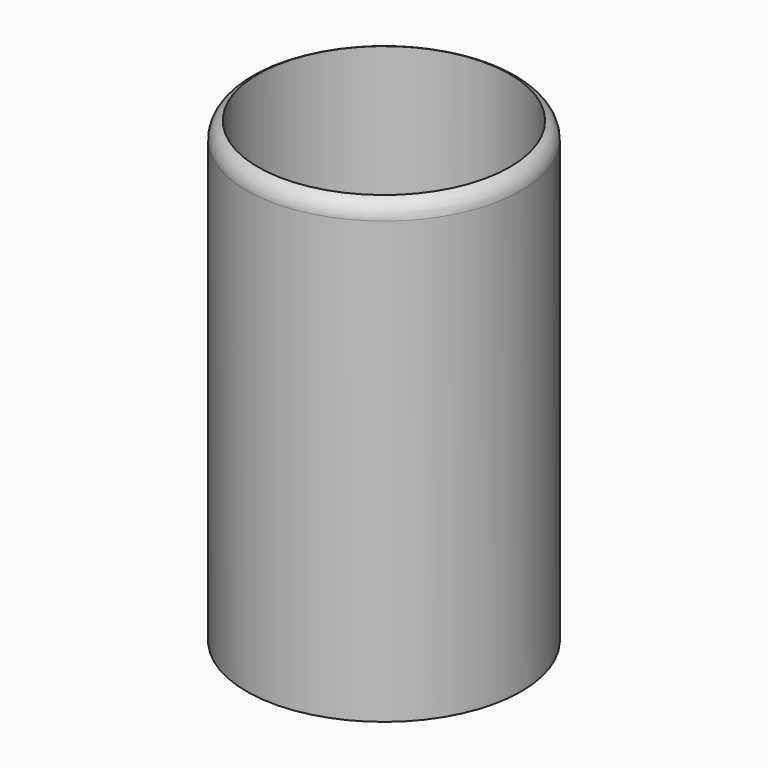
from build123d import *

# Parameters (mm, degrees)
F0_R     = 38.1
F0_R_2   = 34.925
F1_DEPTH = 127
F2_R     = 34.925
F3_DEPTH = 2.54


# Not quite as in the source:
# - a fillet or chamfer that OpenCascade refuses, or shapes differently, is made with other operations: its cross-section is extruded or revolved along the edge and cut away or added


with BuildPart() as f1:
    # F0 (on Top) → F1 (new body)
    with BuildSketch(Plane.XY):
        Circle(F0_R)
        Circle(F0_R_2, mode=Mode.SUBTRACT)
    extrude(amount=F1_DEPTH)

    # F2 (on Top) → F3 (join)
    with BuildSketch(Plane.XY):
        Circle(F2_R)
    extrude(amount=F3_DEPTH)

    # F4: fillet of radius 5.08 on 1 edges, made by hand

    # F4_s1 → F4_t2 (revolve, cut)
    with BuildSketch(Plane.XZ):
        with BuildLine():
            ThreePointArc((38.1, 122.2907139607), (37.2321134838, 125.1305202921), (34.925, 127))
            Line((34.925, 127), (38.1, 127))
            Line((38.1, 127), (38.1, 122.2907139607))
        make_face()
    revolve(axis=Axis((0, 0, 127), (0, 0, 1)), mode=Mode.SUBTRACT)


solid = f1.part
